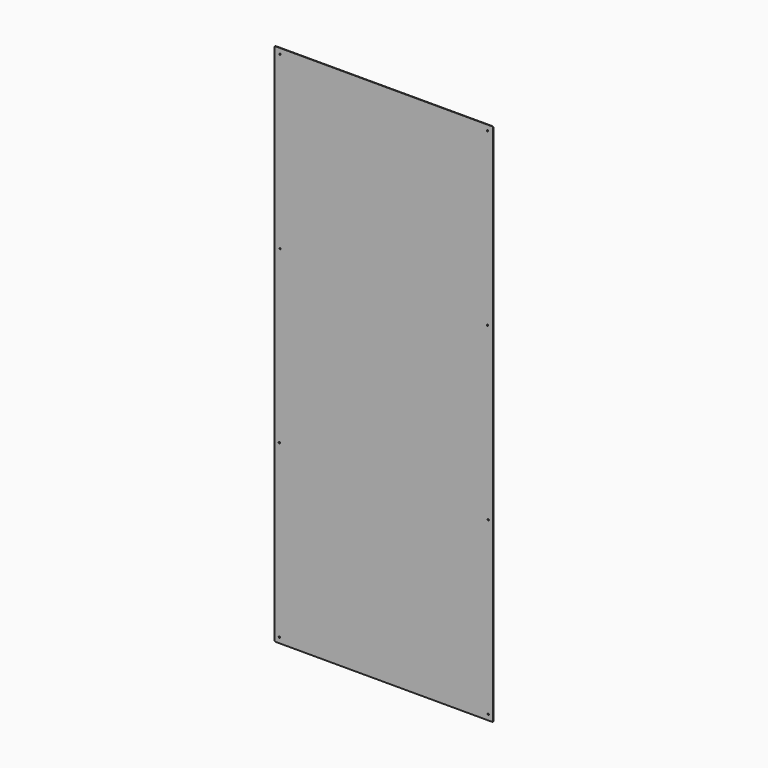
from build123d import *

# Parameters (mm, degrees)
F1_DEPTH = 1.5875
F2_R     = 2.38125
F3_DEPTH = 1.5885


# Not quite as in the source:
# - a length typed as a fraction of an inch, garbled in the dataset ("3 / 203.2 mm" for 3/8 in), is restored


with BuildPart() as f1:
    # F0 (on Front) → F1 (new body)
    with BuildSketch(Plane.XZ):
        with BuildLine():
            Line((-377.825, -914.4), (377.825, -914.4))
            ThreePointArc((377.825, -914.4), (380.0700640303, -913.4700640303), (381, -911.225))
            Line((381, -911.225), (381, 911.225))
            ThreePointArc((381, 911.225), (380.0700640303, 913.4700640303), (377.825, 914.4))
            Line((377.825, 914.4), (-377.825, 914.4))
            ThreePointArc((-377.825, 914.4), (-380.0700640303, 913.4700640303), (-381, 911.225))
            Line((-381, 911.225), (-381, -911.225))
            ThreePointArc((-381, -911.225), (-380.0700640303, -913.4700640303), (-377.825, -914.4))
        make_face()
    extrude(amount=F1_DEPTH)

    # F2 (on face) → F3 (cut, through all)
    with BuildSketch(Plane.XZ.offset(1.5875)):
        with Locations((-361.95, 895.35)):
            Circle(F2_R)
        with Locations((-361.95, 298.44841672)):
            Circle(F2_R)
        with Locations((-364.33125, -298.44841672)):
            Circle(F2_R)
        with Locations((-364.33125, -895.35)):
            Circle(F2_R)
        with Locations((361.95, 895.35)):
            Circle(F2_R)
        with Locations((364.33125, -895.35)):
            Circle(F2_R)
        with Locations((361.95, 298.44841672)):
            Circle(F2_R)
        with Locations((364.33125, -298.44841672)):
            Circle(F2_R)
    extrude(amount=-F3_DEPTH, mode=Mode.SUBTRACT)


solid = f1.part
